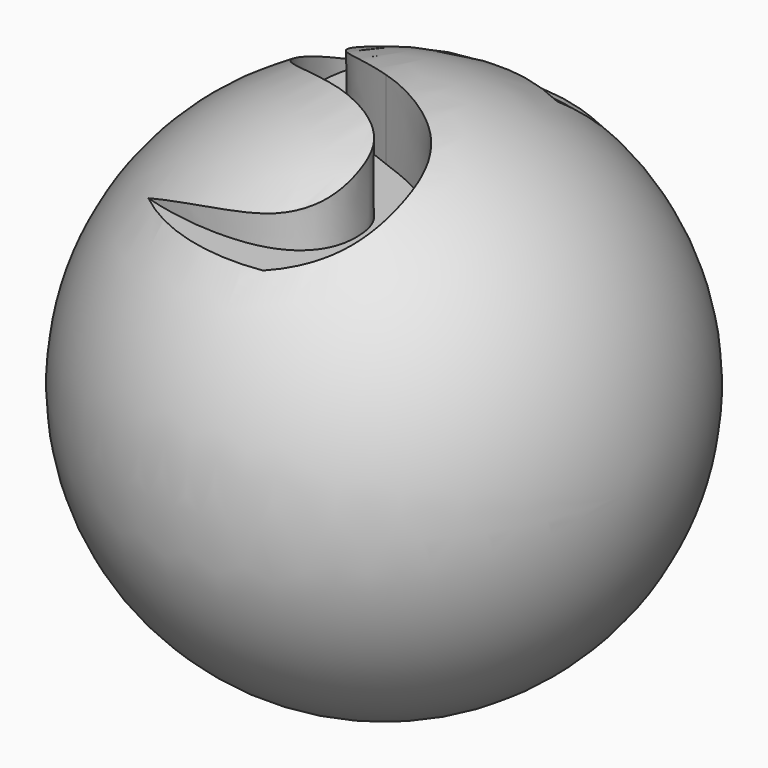
from build123d import *

# Parameters (mm, degrees)
F3_TEXT_SIZE = 98.9932929062
F4_DEPTH     = 15


# Not quite as in the source:
# - Text() gives the source's letters only with a copy of the font that has no kerning and outlines rounded to 1/6400 em; it was checked with that copy


with BuildPart() as f1:
    # F0 (on Top) → F1 (revolve)
    with BuildSketch(Plane.XY):
        with BuildLine():
            ThreePointArc((-50, 0), (0, -50), (50, 0))
            Line((50, 0), (-50, 0))
        make_face()
    revolve(axis=Axis((-0.9944587946, 0, 0), (-1, 0, 0)))

    # F3 (on offset) → F4 (cut)
    with BuildSketch(Plane.XY.offset(50)):
        with Locations((-31.8669974804, -36.4188961685)):
            Text('S', F3_TEXT_SIZE, font='Open Sans', text_align=(TextAlign.LEFT, TextAlign.BOTTOM))
    extrude(amount=-F4_DEPTH, mode=Mode.SUBTRACT)


solid = f1.part
